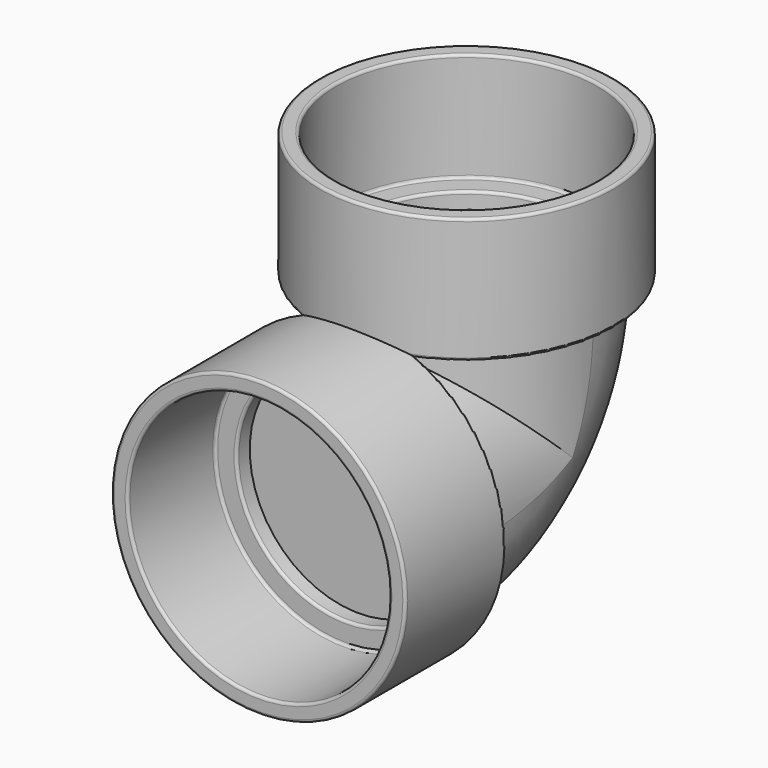
from build123d import *

# Parameters (mm, degrees)
F1_DEPTH     = 46.5
F2_T1_DEPTH  = 59.625
F2_T3_DEPTH  = 59.625
F2_T6_ANGLE  = 228.8189583237
F2_T8_ANGLE  = 228.8189583237
F2_T13_DEPTH = 117.75
F2_T17_DEPTH = 117.75
F2_T24_DEPTH = 117.75
F2_T28_DEPTH = 117.75
F3_R         = 24
F3_R_2       = 20
F5_DEPTH     = 3
F3_R_3       = 27
F6_DEPTH     = 23
F4_R         = 24
F4_R_2       = 20
F7_DEPTH     = 3
F4_R_3       = 27
F8_DEPTH     = 23
F9_R         = 0.5


# Not quite as in the source:
# - a fillet or chamfer that OpenCascade refuses, or shapes differently, is made with other operations: its cross-section is extruded or revolved along the edge and cut away or added
# - a feature names something its author has since deleted; it is built from what else it names


with BuildPart() as f1:
    # F0 (on Right) → F1 (new body)
    with BuildSketch(Plane.YZ):
        with BuildLine():
            Line((-22.5, 24.75), (-22.5, 23.25))
            Line((-22.5, 23.25), (-24, 23.25))
            Line((-24, 23.25), (-24, -23.25))
            ThreePointArc((-24, -23.25), (9.941125497, -9.191125497), (24, 24.75))
            Line((24, 24.75), (-22.5, 24.75))
        make_face()
    extrude(amount=F1_DEPTH)

    # F2: fillet of radius 23.25 on 6 edges, made by hand

    # F2_s2 → F2_t1 (cut)
    with BuildSketch(Plane.XY.offset(23.25)):
        with BuildLine():
            ThreePointArc((23.25, -22.5), (39.6902326626, -15.6902326626), (46.5, 0.75))
            Line((46.5, 0.75), (46.5, -22.5))
            Line((46.5, -22.5), (23.25, -22.5))
        make_face()
        with BuildLine():
            ThreePointArc((23.25, -22.5), (6.8097673374, -15.6902326626), (0, 0.75))
            Line((0, 0.75), (0, -22.5))
            Line((0, -22.5), (23.25, -22.5))
        make_face()
    extrude(amount=F2_T1_DEPTH, mode=Mode.SUBTRACT)

    # F2_s4 → F2_t3 (cut)
    with BuildSketch(Plane.XZ.offset(22.5)):
        with BuildLine():
            ThreePointArc((23.25, 23.25), (39.6902326626, 16.4402326626), (46.5, 0))
            Line((46.5, 0), (46.5, 23.25))
            Line((46.5, 23.25), (23.25, 23.25))
        make_face()
        with BuildLine():
            ThreePointArc((23.25, 23.25), (6.8097673374, 16.4402326626), (0, 0))
            Line((0, 0), (0, 23.25))
            Line((0, 23.25), (23.25, 23.25))
        make_face()
    extrude(amount=F2_T3_DEPTH, mode=Mode.SUBTRACT)

    # F2_s5 → F2_t6 (revolve, cut)
    with BuildSketch(Plane(origin=(0, -11.1166068872, 29.5901166597), x_dir=(1, 0, 0), z_dir=(0, -0.3516867795, 0.9361177325))):
        with BuildLine():
            ThreePointArc((23.25, -61.7625777883), (6.8097673374, -54.9528104509), (0, -38.5125777883))
            Line((0, -38.5125777883), (0, -61.7625777883))
            Line((0, -61.7625777883), (23.25, -61.7625777883))
        make_face()
    revolve(axis=Axis((0, -24, 24.75), (1, 0, 0)), revolution_arc=F2_T6_ANGLE, mode=Mode.SUBTRACT)

    # F2_s7 → F2_t8 (revolve, cut)
    with BuildSketch(Plane(origin=(0, -11.1166068872, 29.5901166597), x_dir=(1, 0, 0), z_dir=(0, -0.3516867795, 0.9361177325))):
        with BuildLine():
            ThreePointArc((23.25, -61.7625777883), (39.6902326626, -54.9528104509), (46.5, -38.5125777883))
            Line((46.5, -38.5125777883), (46.5, -61.7625777883))
            Line((46.5, -61.7625777883), (23.25, -61.7625777883))
        make_face()
    revolve(axis=Axis((46.5, -24, 24.75), (1, 0, 0)), revolution_arc=F2_T8_ANGLE, mode=Mode.SUBTRACT)


with BuildPart() as f2_tool11:
    # F2_s12 → F2_t13 (new body)
    with BuildSketch(Plane.XY.offset(82.875)):
        with BuildLine():
            ThreePointArc((23.25, -22.5), (39.6902326626, -15.6902326626), (46.5, 0.75))
            Line((46.5, 0.75), (46.5, -22.5))
            Line((46.5, -22.5), (23.25, -22.5))
        make_face()
    extrude(amount=-F2_T13_DEPTH)

    split(bisect_by=Plane.XY.offset(23.25), keep=Keep.BOTTOM)


with BuildPart() as f2_tool15:
    # F2_s16 → F2_t17 (new body)
    with BuildSketch(Plane.XZ.offset(-35.625)):
        with BuildLine():
            ThreePointArc((23.25, 23.25), (39.6902326626, 16.4402326626), (46.5, 0))
            Line((46.5, 0), (46.5, 23.25))
            Line((46.5, 23.25), (23.25, 23.25))
        make_face()
    extrude(amount=F2_T17_DEPTH)

    split(bisect_by=Plane.XZ.offset(22.5), keep=Keep.BOTTOM)


with BuildPart() as f2_tool11_1:
    add(f2_tool11.part)

    # F2_t19: intersect F2_tool15
    add(f2_tool15.part, mode=Mode.INTERSECT)


with BuildPart() as f1_1:
    add(f1.part)

    # F2_t9: cut F2_tool11
    add(f2_tool11_1.part, mode=Mode.SUBTRACT)


with BuildPart() as f2_tool22:
    # F2_s23 → F2_t24 (new body)
    with BuildSketch(Plane.XY.offset(82.875)):
        with BuildLine():
            ThreePointArc((23.25, -22.5), (6.8097673374, -15.6902326626), (0, 0.75))
            Line((0, 0.75), (0, -22.5))
            Line((0, -22.5), (23.25, -22.5))
        make_face()
    extrude(amount=-F2_T24_DEPTH)

    split(bisect_by=Plane.XY.offset(23.25), keep=Keep.BOTTOM)


with BuildPart() as f2_tool26:
    # F2_s27 → F2_t28 (new body)
    with BuildSketch(Plane.XZ.offset(-35.625)):
        with BuildLine():
            ThreePointArc((23.25, 23.25), (6.8097673374, 16.4402326626), (0, 0))
            Line((0, 0), (0, 23.25))
            Line((0, 23.25), (23.25, 23.25))
        make_face()
    extrude(amount=F2_T28_DEPTH)

    split(bisect_by=Plane.XZ.offset(22.5), keep=Keep.BOTTOM)


with BuildPart() as f2_tool22_1:
    add(f2_tool22.part)

    # F2_t30: intersect F2_tool26
    add(f2_tool26.part, mode=Mode.INTERSECT)


with BuildPart() as f1_2:
    add(f1_1.part)

    # F2_t20: cut F2_tool22
    add(f2_tool22_1.part, mode=Mode.SUBTRACT)

    # F3 (on face) → F5 (join)
    with BuildSketch(Plane.XY.offset(24.75)):
        with Locations((23.25, 0.75)):
            Circle(F3_R)
        with BuildLine():
            ThreePointArc((46.5, 0.75), (39.6902326626, -15.6902326626), (23.25, -22.5))
            ThreePointArc((23.25, -22.5), (6.8097673374, -15.6902326626), (0, 0.75))
            ThreePointArc((0, 0.75), (6.8097673374, 17.1902326626), (23.25, 24))
            ThreePointArc((23.25, 24), (39.6902326626, 17.1902326626), (46.5, 0.75))
        make_face(mode=Mode.SUBTRACT)
        with BuildLine():
            ThreePointArc((0, 0.75), (6.8097673374, -15.6902326626), (23.25, -22.5))
            ThreePointArc((23.25, -22.5), (39.6902326626, -15.6902326626), (46.5, 0.75))
            ThreePointArc((46.5, 0.75), (39.6902326626, 17.1902326626), (23.25, 24))
            ThreePointArc((23.25, 24), (6.8097673374, 17.1902326626), (0, 0.75))
        make_face()
        with Locations((23.25, 0.75)):
            Circle(F3_R_2, mode=Mode.SUBTRACT)
    extrude(amount=F5_DEPTH)

    # F3 (on face) → F6 (join)
    with BuildSketch(Plane.XY.offset(24.75)):
        with Locations((23.25, 0.75)):
            Circle(F3_R_3)
        with Locations((23.25, 0.75)):
            Circle(F3_R, mode=Mode.SUBTRACT)
    extrude(amount=F6_DEPTH)

    # F4 (on face) → F7 (join)
    with BuildSketch(Plane.XZ.offset(24)):
        with Locations((23.25, 0)):
            Circle(F4_R)
        with BuildLine():
            ThreePointArc((46.5, 0), (39.6902326626, -16.4402326626), (23.25, -23.25))
            ThreePointArc((23.25, -23.25), (6.8097673374, -16.4402326626), (0, 0))
            ThreePointArc((0, 0), (6.8097673374, 16.4402326626), (23.25, 23.25))
            ThreePointArc((23.25, 23.25), (39.6902326626, 16.4402326626), (46.5, 0))
        make_face(mode=Mode.SUBTRACT)
        with BuildLine():
            ThreePointArc((0, 0), (6.8097673374, -16.4402326626), (23.25, -23.25))
            ThreePointArc((23.25, -23.25), (39.6902326626, -16.4402326626), (46.5, 0))
            ThreePointArc((46.5, 0), (39.6902326626, 16.4402326626), (23.25, 23.25))
            ThreePointArc((23.25, 23.25), (6.8097673374, 16.4402326626), (0, 0))
        make_face()
        with Locations((23.25, 0)):
            Circle(F4_R_2, mode=Mode.SUBTRACT)
    extrude(amount=F7_DEPTH)

    # F4 (on face) → F8 (join)
    with BuildSketch(Plane.XZ.offset(24)):
        with Locations((23.25, 0)):
            Circle(F4_R_3)
        with Locations((23.25, 0)):
            Circle(F4_R, mode=Mode.SUBTRACT)
    extrude(amount=F8_DEPTH)

    # F9
    f9_edges = [f1_2.edges().sort_by_distance(p)[0] for p in [
        (8.457211, -24, -22.587018),
        (8.457211, 23.337018, 24.75),
        (-3.75, -47, 0),
        (-0.75, -47, 0),
        (-3.75, 0.75, 47.75),
        (-0.75, 0.75, 47.75),
        (-0.75, 0.75, 27.75),
        (3.25, 0.75, 27.75),
        (3.25, -27, 0),
        (-0.75, -27, 0),
    ]]
    fillet(f9_edges, radius=F9_R)


solid = f1_2.part
